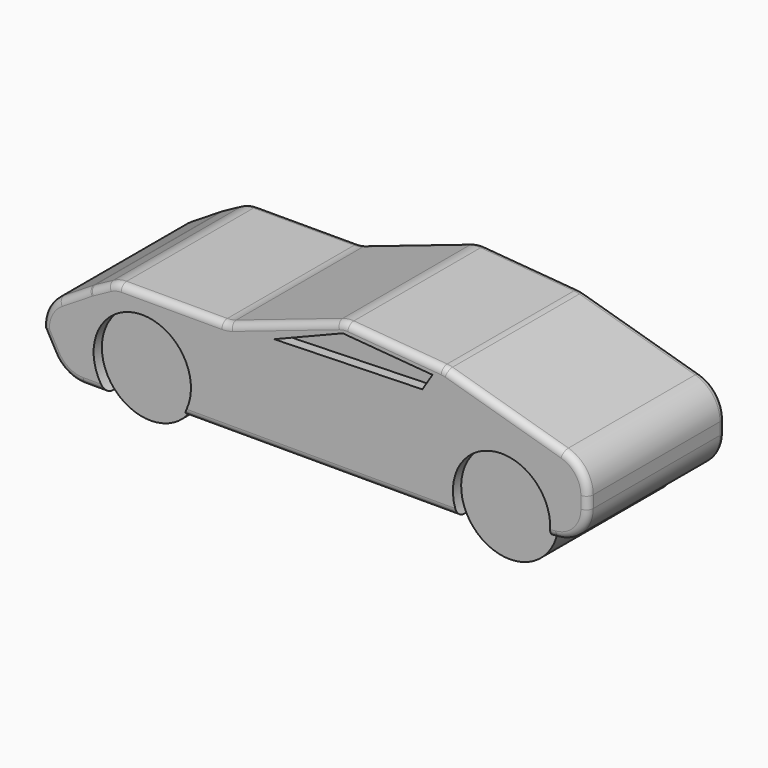
from build123d import *

# Parameters (mm, degrees)
F1_DEPTH    = 25
F2_T1_DEPTH = 25
F2_T3_DEPTH = 33.2865856195
F2_T5_DEPTH = 35.1375068729
F2_T7_DEPTH = 26.2439265081
F2_T9_DEPTH = 29.0269565503
F3_T1_DEPTH = 64.9996021944
F3_T3_DEPTH = 54.4201853444
F3_T5_DEPTH = 62.5652900515
F3_T7_DEPTH = 70.9771112235
F4_R        = 14.1322148091
F5_DEPTH    = 3
F6_R        = 2


# Not quite as in the source:
# - a fillet or chamfer that OpenCascade refuses, or shapes differently, is made with other operations: its cross-section is extruded or revolved along the edge and cut away or added


with BuildPart() as f1:
    # F0 (on Front) → F1 (new body)
    with BuildSketch(Plane.XZ):
        with BuildLine():
            Line((-81.2098225326, -15.6771827859), (-68.6711987798, -15.6771827859))
            ThreePointArc((-68.6711987798, -15.6771827859), (-57.1419560716, -20.274533801), (-46.4318082669, -14.0014318744))
            Line((-46.4318082669, -14.0014318744), (33.4813362922, -14.0014318744))
            ThreePointArc((33.4813362922, -14.0014318744), (48.0187694937, -21.717844135), (60.0034566781, -10.4374516171))
            Line((60.0034566781, -10.4374516171), (71.1715072393, -9.4995843247))
            Line((71.1715072393, -9.4995843247), (71.1715072393, 10.7058854774))
            Line((71.1715072393, 10.7058854774), (29.5542683452, 22.7688532323))
            Line((29.5542683452, 22.7688532323), (0, 25.1814462245))
            Line((0, 25.1814462245), (-33.7763093412, 13.7216281146))
            Line((-33.7763093412, 13.7216281146), (-66.3463175297, 13.7216281146))
            Line((-66.3463175297, 13.7216281146), (-73.5840946436, 9.8011633381))
            Line((-73.5840946436, 9.8011633381), (-89.2659574747, 0))
            Line((-89.2659574747, 0), (-87.1549323201, -4.9759717658))
            Line((-87.1549323201, -4.9759717658), (-81.2098225326, -15.6771827859))
        make_face()
    extrude(amount=F1_DEPTH)

    # F2: fillet of radius 8 on 5 edges, made by hand

    # F2_s2 → F2_t1 (join)
    with BuildSketch(Plane.XZ):
        with BuildLine():
            ThreePointArc((-32.5261230106, 14.1457984349), (-33.7939263524, 13.8283829823), (-35.0964935411, 13.7216281146))
            Line((-35.0964935411, 13.7216281146), (-33.7763093412, 13.7216281146))
            Line((-33.7763093412, 13.7216281146), (-32.5261230106, 14.1457984349))
        make_face()
    extrude(amount=F2_T1_DEPTH)

    # F2_s4 → F2_t3 (cut)
    with BuildSketch(Plane.XZ.offset(-4.1432928098)):
        with BuildLine():
            ThreePointArc((1.6518224825, 25.0466035919), (0.0208109602, 25.012860503), (-1.569444032, 24.6489563376))
            Line((-1.569444032, 24.6489563376), (0, 25.1814462245))
            Line((0, 25.1814462245), (1.6518224825, 25.0466035919))
        make_face()
    extrude(amount=F2_T3_DEPTH, mode=Mode.SUBTRACT)

    # F2_s6 → F2_t5 (cut)
    with BuildSketch(Plane.XZ.offset(-5.0687534365)):
        with BuildLine():
            ThreePointArc((-64.3188161551, 13.7216281146), (-66.284181416, 13.4764549593), (-68.1290829763, 12.7559629624))
            Line((-68.1290829763, 12.7559629624), (-66.3463175297, 13.7216281146))
            Line((-66.3463175297, 13.7216281146), (-64.3188161551, 13.7216281146))
        make_face()
    extrude(amount=F2_T5_DEPTH, mode=Mode.SUBTRACT)

    # F2_s8 → F2_t7 (cut)
    with BuildSketch(Plane.XZ.offset(-0.6219632541)):
        with BuildLine():
            ThreePointArc((-73.365339754, 9.9196556357), (-73.5821478307, 9.7978216209), (-73.7950641631, 9.669307401))
            Line((-73.7950641631, 9.669307401), (-73.5840946436, 9.8011633381))
            Line((-73.5840946436, 9.8011633381), (-73.365339754, 9.9196556357))
        make_face()
    extrude(amount=F2_T7_DEPTH, mode=Mode.SUBTRACT)

    # F2_s10 → F2_t9 (cut)
    with BuildSketch(Plane.XZ.offset(-2.0134782752)):
        with BuildLine():
            ThreePointArc((30.3278196103, 22.544635475), (29.5469574945, 22.7290808385), (28.751547216, 22.8343814784))
            Line((28.751547216, 22.8343814784), (29.5542683452, 22.7688532323))
            Line((29.5542683452, 22.7688532323), (30.3278196103, 22.544635475))
        make_face()
    extrude(amount=F2_T9_DEPTH, mode=Mode.SUBTRACT)

    # F3: fillet of radius 10 on 4 edges, made by hand

    # F3_s2 → F3_t1 (cut)
    with BuildSketch(Plane.XZ.offset(-19.9998010972)):
        with BuildLine():
            ThreePointArc((-87.1549323201, -4.9759717658), (-86.1010433194, 0.2823042988), (-82.4820383293, 4.239949063))
            Line((-82.4820383293, 4.239949063), (-89.2659574747, 0))
            Line((-89.2659574747, 0), (-87.1549323201, -4.9759717658))
        make_face()
    extrude(amount=F3_T1_DEPTH, mode=Mode.SUBTRACT)

    # F3_s4 → F3_t3 (cut)
    with BuildSketch(Plane.XZ.offset(-14.7100926722)):
        with BuildLine():
            ThreePointArc((-75.3257854638, -15.6771827859), (-80.3970650538, -14.2958905382), (-84.0673608071, -10.5336074498))
            Line((-84.0673608071, -10.5336074498), (-81.2098225326, -15.6771827859))
            Line((-81.2098225326, -15.6771827859), (-75.3257854638, -15.6771827859))
        make_face()
    extrude(amount=F3_T3_DEPTH, mode=Mode.SUBTRACT)

    # F3_s6 → F3_t5 (cut)
    with BuildSketch(Plane.XZ.offset(-18.7826450258)):
        with BuildLine():
            ThreePointArc((63.9554677121, 12.7974911304), (69.1664933159, 9.1995068855), (71.1715072393, 3.1928274671))
            Line((71.1715072393, 3.1928274671), (71.1715072393, 10.7058854774))
            Line((71.1715072393, 10.7058854774), (63.9554677121, 12.7974911304))
        make_face()
    extrude(amount=F3_T5_DEPTH, mode=Mode.SUBTRACT)

    # F3_s8 → F3_t7 (cut)
    with BuildSketch(Plane.XZ.offset(-22.9885556118)):
        with BuildLine():
            ThreePointArc((71.1715072393, -0.30416208), (68.532496131, -7.0729021797), (62.0083387319, -10.2690862168))
            Line((62.0083387319, -10.2690862168), (71.1715072393, -9.4995843247))
            Line((71.1715072393, -9.4995843247), (71.1715072393, -0.30416208))
        make_face()
    extrude(amount=F3_T7_DEPTH, mode=Mode.SUBTRACT)

    # F4 (on face) → F5 (cut)
    with BuildSketch(Plane.XZ.offset(25)):
        Polygon((0.0208109602, 22.1540294588), (-19.880797714, 14.1719523817), (23.1445431709, 15.3400599957), (26.0648149997, 20.0124960393), align=None)
        with Locations((-58.2038164139, -6.1822682619)):
            Circle(F4_R)
        with Locations((46.1366328286, -7.7115220987)):
            Circle(F4_R)
    extrude(amount=-F5_DEPTH, mode=Mode.SUBTRACT)

    # F6
    f6_edges = [f1.edges().sort_by_distance(p)[0] for p in [
        (-71.998492, -25, -15.677183),
        (-86.101043, -25, 0.282304),
        (-78.138551, -25, 6.954628),
        (-6.475236, -25, -14.001432),
        (-80.397065, -25, -14.295891),
        (-85.611147, -25, -7.75479),
        (-73.582148, -25, 9.797822),
        (-70.747211, -25, 11.337809),
        (-66.284181, -25, 13.476455),
        (-49.707655, -25, 13.721628),
        (-33.793926, -25, 13.828383),
        (-17.047784, -25, 19.397377),
        (0.020811, -25, 25.012861),
        (15.201685, -25, 23.940493),
        (29.546957, -25, 22.729081),
        (47.141644, -25, 17.671063),
        (69.166493, -25, 9.199507),
        (71.171507, -25, 1.444333),
        (68.532496, -25, -7.072902),
        (61.005898, -25, -10.353269),
    ]]
    fillet(f6_edges, radius=F6_R)

    # F7: F1 across plane


with BuildPart() as f1_1:
    add(f1.part)
    add(f1.part.mirror(Plane.XZ))


solid = f1_1.part
